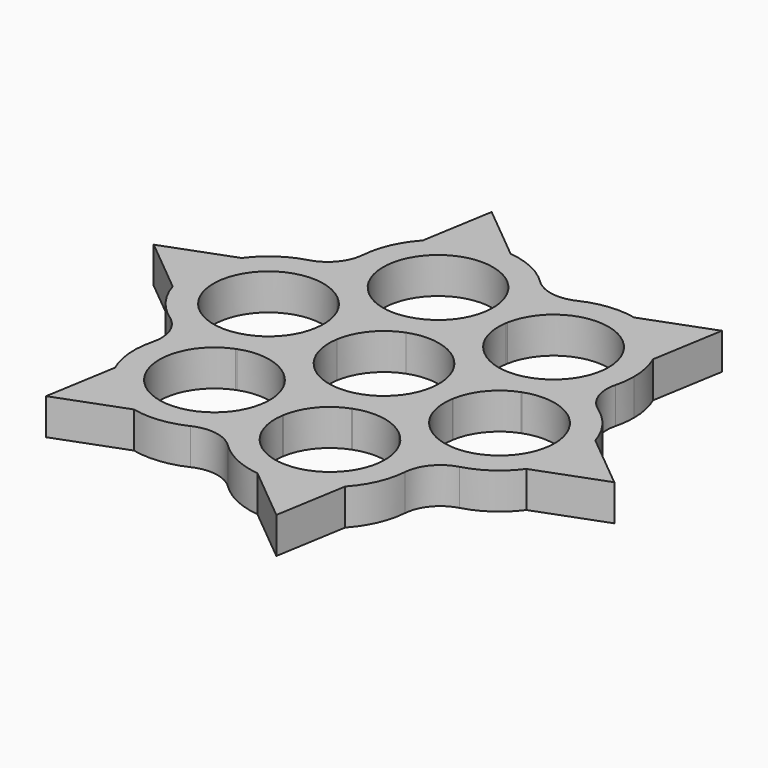
from build123d import *

# Parameters (mm, degrees)
F2_DEPTH    = 7.239
F3_DEPTH    = 7.239
F4_T1_DEPTH = 7.239
F5_R        = 7.62


# Not quite as in the source:
# - a fillet or chamfer that OpenCascade refuses, or shapes differently, is made with other operations: its cross-section is extruded or revolved along the edge and cut away or added


with BuildPart() as f2:
    # F0 (on Top) → F2 (new body)
    with BuildSketch(Plane.XY):
        with BuildLine():
            ThreePointArc((6.9968392918, 8.4855549709), (9.9476892075, 4.6908296356), (10.9982, 0))
            ThreePointArc((10.9982, 0), (10.9603663805, -0.9114669745), (10.8471258159, -1.8166630875))
            Line((10.8471258159, -1.8166630875), (15.8573455923, -2.6557684397))
            ThreePointArc((15.8573455923, -2.6557684397), (16.0228912675, -1.3324678865), (16.0782, 0))
            ThreePointArc((16.0782, 0), (14.542464823, 6.8574945943), (10.2286357315, 12.4049798997))
            Line((10.2286357315, 12.4049798997), (6.9968392918, 8.4855549709))
        make_face()
        with BuildLine():
            ThreePointArc((-3.8502865241, 10.3022180584), (1.8166630875, 10.8471258159), (6.9968392918, 8.4855549709))
            Line((6.9968392918, 8.4855549709), (10.2286357315, 12.4049798997))
            ThreePointArc((10.2286357315, 12.4049798997), (2.6557684397, 15.8573455923), (-5.6287098609, 15.0607483394))
            Line((-5.6287098609, 15.0607483394), (-3.8502865241, 10.3022180584))
        make_face()
        with BuildLine():
            Line((15.8573455923, -2.6557684397), (10.8471258159, -1.8166630875))
            ThreePointArc((10.8471258159, -1.8166630875), (8.4855549709, -6.9968392918), (3.8502865241, -10.3022180584))
            Line((3.8502865241, -10.3022180584), (5.6287098609, -15.0607483394))
            ThreePointArc((5.6287098609, -15.0607483394), (12.4049798997, -10.2286357315), (15.8573455923, -2.6557684397))
        make_face()
        with BuildLine():
            ThreePointArc((-10.8471258159, 1.8166630875), (-8.4855549709, 6.9968392918), (-3.8502865241, 10.3022180584))
            Line((-3.8502865241, 10.3022180584), (-5.6287098609, 15.0607483394))
            ThreePointArc((-5.6287098609, 15.0607483394), (-12.4049798997, 10.2286357315), (-15.8573455923, 2.6557684397))
            Line((-15.8573455923, 2.6557684397), (-10.8471258159, 1.8166630875))
        make_face()
        with BuildLine():
            Line((5.6287098609, -15.0607483394), (3.8502865241, -10.3022180584))
            ThreePointArc((3.8502865241, -10.3022180584), (-1.8166630875, -10.8471258159), (-6.9968392918, -8.4855549709))
            Line((-6.9968392918, -8.4855549709), (-10.2286357315, -12.4049798997))
            ThreePointArc((-10.2286357315, -12.4049798997), (-2.6557684397, -15.8573455923), (5.6287098609, -15.0607483394))
        make_face()
        with BuildLine():
            ThreePointArc((-6.9968392918, -8.4855549709), (-10.3022180584, -3.8502865241), (-10.8471258159, 1.8166630875))
            Line((-10.8471258159, 1.8166630875), (-15.8573455923, 2.6557684397))
            ThreePointArc((-15.8573455923, 2.6557684397), (-15.0607483394, -5.6287098609), (-10.2286357315, -12.4049798997))
            Line((-10.2286357315, -12.4049798997), (-6.9968392918, -8.4855549709))
        make_face()
    extrude(amount=F2_DEPTH)

    # F1 (on Top) → F3 (join)
    with BuildSketch(Plane.XY):
        with BuildLine():
            ThreePointArc((22.9514427755, 5.8656594668), (33.016468503, 4.5341364803), (37.7025851565, -4.4724170818))
            ThreePointArc((37.7025851565, -4.4724170818), (31.4379323636, -14.3998504902), (19.7807553883, -13.017810816))
            ThreePointArc((19.7807553883, -13.017810816), (22.8084512552, -16.3716447193), (24.7834468313, -20.4354528579))
            ThreePointArc((24.7834468313, -20.4354528579), (33.1080256386, -19.2203628308), (39.6794010209, -13.9675462837))
            ThreePointArc((39.6794010209, -13.9675462837), (41.9871109493, -9.4670950078), (42.7825851565, -4.4724170818))
            ThreePointArc((42.7825851565, -4.4724170818), (42.6022135722, -2.0708411606), (42.0651457783, 0.2768511103))
            ThreePointArc((42.0651457783, 0.2768511103), (37.5638328916, 7.3842650059), (30.0893074574, 11.2454331611))
            ThreePointArc((30.0893074574, 11.2454331611), (26.9017291405, 8.0495671456), (22.9514427755, 5.8656594668))
        make_face()
        with BuildLine():
            ThreePointArc((22.7561188104, 5.7926497032), (22.8536077582, 5.829617507), (22.9514427755, 5.8656594668))
            ThreePointArc((22.9514427755, 5.8656594668), (26.9017291405, 8.0495671456), (30.0893074574, 11.2454331611))
            ThreePointArc((30.0893074574, 11.2454331611), (25.5869892554, 11.5669077681), (21.1727380342, 10.624251271))
            ThreePointArc((21.1727380342, 10.624251271), (21.0752490864, 10.5872834672), (20.9774140691, 10.5512415074))
            ThreePointArc((20.9774140691, 10.5512415074), (17.0271277041, 8.3673338285), (13.8395493871, 5.1714678131))
            ThreePointArc((13.8395493871, 5.1714678131), (18.3418675892, 4.849993206), (22.7561188104, 5.7926497032))
        make_face()
        with BuildLine():
            ThreePointArc((24.7834468313, -20.4354528579), (22.8084512552, -16.3716447193), (19.7807553883, -13.017810816))
            ThreePointArc((19.7807553883, -13.017810816), (19.707218441, -12.957702062), (19.6342033145, -12.8969605092))
            ThreePointArc((19.6342033145, -12.8969605092), (15.7650750743, -10.5635101082), (11.3994817591, -9.3987186595))
            ThreePointArc((11.3994817591, -9.3987186595), (13.3744773351, -13.4625267981), (16.402173202, -16.8163607014))
            ThreePointArc((16.402173202, -16.8163607014), (16.4757101493, -16.8764694554), (16.5487252758, -16.9372110082))
            ThreePointArc((16.5487252758, -16.9372110082), (20.417853516, -19.2706614092), (24.7834468313, -20.4354528579))
        make_face()
        with BuildLine():
            ThreePointArc((21.1727380342, 10.624251271), (25.5869892554, 11.5669077681), (30.0893074574, 11.2454331611))
            ThreePointArc((30.0893074574, 11.2454331611), (32.4781911968, 15.8067442605), (33.302671688, 20.8893180559))
            ThreePointArc((33.302671688, 20.8893180559), (32.9570434325, 24.2051439777), (31.9350184005, 27.3784112637))
            ThreePointArc((31.9350184005, 27.3784112637), (27.4531526953, 33.294260623), (20.7917042689, 36.566797667))
            ThreePointArc((20.7917042689, 36.566797667), (12.3866178149, 36.2224092362), (5.3058447451, 31.6807427551))
            ThreePointArc((5.3058447451, 31.6807427551), (6.2730175907, 28.5865669578), (6.5998373584, 25.3612706897))
            ThreePointArc((6.5998373584, 25.3612706897), (6.5505250686, 24.1029885217), (6.4028906835, 22.852424727))
            ThreePointArc((6.4028906835, 22.852424727), (18.2099895812, 31.8432743148), (28.222671688, 20.8893180559))
            ThreePointArc((28.222671688, 20.8893180559), (26.2904582909, 14.6628993296), (21.1727380342, 10.624251271))
        make_face()
        with BuildLine():
            ThreePointArc((25.5567434338, -25.3617544356), (25.3622428304, -22.8684416359), (24.7834468313, -20.4354528579))
            ThreePointArc((24.7834468313, -20.4354528579), (20.417853516, -19.2706614092), (16.5487252758, -16.9372110082))
            ThreePointArc((16.5487252758, -16.9372110082), (19.4464839727, -20.7141136736), (20.4767434338, -25.3617544356))
            ThreePointArc((20.4767434338, -25.3617544356), (8.6144991811, -36.3259612364), (-1.3838939013, -23.6390071003))
            ThreePointArc((-1.3838939013, -23.6390071003), (-2.7742058336, -27.9382250388), (-5.3058324685, -31.6808322496))
            ThreePointArc((-5.3058324685, -31.6808322496), (-0.0911857517, -38.2818472587), (7.7431459541, -41.3460251674))
            ThreePointArc((7.7431459541, -41.3460251674), (15.1072895917, -40.4224892095), (21.2720483325, -36.289780673))
            ThreePointArc((21.2720483325, -36.289780673), (24.4472916397, -31.2307485904), (25.5567434338, -25.3617544356))
        make_face()
        with BuildLine():
            Line((53.2084477738, -8.9112843948), (42.0651457783, 0.2768511103))
            ThreePointArc((42.0651457783, 0.2768511103), (42.6022135722, -2.0708411606), (42.7825851565, -4.4724170818))
            ThreePointArc((42.7825851565, -4.4724170818), (41.9871109493, -9.4670950078), (39.6794010209, -13.9675462837))
            Line((39.6794010209, -13.9675462837), (53.2084477738, -8.9112843948))
        make_face()
        with BuildLine():
            ThreePointArc((1.3432183629, 23.3981640186), (1.2689892456, 18.9066190694), (2.4402643012, 14.5698459906))
            ThreePointArc((2.4402643012, 14.5698459906), (4.9605713467, 18.2883858101), (6.3537578179, 22.5590435404))
            ThreePointArc((6.3537578179, 22.5590435404), (6.3773323249, 22.7059002526), (6.4028906835, 22.852424727))
            ThreePointArc((6.4028906835, 22.852424727), (6.5505250686, 24.1029885217), (6.5998373584, 25.3612706897))
            ThreePointArc((6.5998373584, 25.3612706897), (6.2730175907, 28.5865669578), (5.3058447451, 31.6807427551))
            ThreePointArc((5.3058447451, 31.6807427551), (2.7855376997, 27.9622029355), (1.3923512285, 23.6915452052))
            ThreePointArc((1.3923512285, 23.6915452052), (1.3687767215, 23.544688493), (1.3432183629, 23.3981640186))
        make_face()
        with BuildLine():
            ThreePointArc((20.7917042689, 36.566797667), (27.4531526953, 33.294260623), (31.9350184005, 27.3784112637))
            Line((31.9350184005, 27.3784112637), (34.3206748537, 41.6230759294))
            Line((34.3206748537, 41.6230759294), (20.7917042689, 36.566797667))
        make_face()
        with BuildLine():
            ThreePointArc((-1.1472239849, -20.8904729728), (-1.4740007496, -17.6653867253), (-2.4410480826, -14.5713951588))
            ThreePointArc((-2.4410480826, -14.5713951588), (-4.9726747175, -18.3140023695), (-6.3629866498, -22.6132203081))
            ThreePointArc((-6.3629866498, -22.6132203081), (-6.3782276583, -22.7067149977), (-6.3942733749, -22.800074948))
            ThreePointArc((-6.3942733749, -22.800074948), (-6.4802418832, -27.317690643), (-5.3058324685, -31.6808322496))
            ThreePointArc((-5.3058324685, -31.6808322496), (-2.7742058336, -27.9382250388), (-1.3838939013, -23.6390071003))
            ThreePointArc((-1.3838939013, -23.6390071003), (-1.3686528928, -23.5455124107), (-1.3526071762, -23.4521524604))
            ThreePointArc((-1.3526071762, -23.4521524604), (-1.1986520321, -22.1754227824), (-1.1472239849, -20.8904729728))
        make_face()
        with BuildLine():
            Line((18.8864028853, -50.5343796221), (21.2720483325, -36.289780673))
            ThreePointArc((21.2720483325, -36.289780673), (15.1072895917, -40.4224892095), (7.7431459541, -41.3460251674))
            Line((7.7431459541, -41.3460251674), (18.8864028853, -50.5343796221))
        make_face()
        with BuildLine():
            ThreePointArc((-19.5826320581, 12.8547821817), (-15.7335197941, 10.5497372026), (-11.3973465236, 9.3979998437))
            ThreePointArc((-11.3973465236, 9.3979998437), (-13.3543168627, 13.4352222389), (-16.3506403955, 16.7745249899))
            ThreePointArc((-16.3506403955, 16.7745249899), (-16.4751157371, 16.8756446455), (-16.5981033888, 16.9785685637))
            ThreePointArc((-16.5981033888, 16.9785685637), (-20.4472156527, 19.2836135428), (-24.7833889233, 20.4353509017))
            ThreePointArc((-24.7833889233, 20.4353509017), (-22.8264185841, 16.3981285065), (-19.8300950513, 13.0588257555))
            ThreePointArc((-19.8300950513, 13.0588257555), (-19.7056197098, 12.9577060999), (-19.5826320581, 12.8547821817))
        make_face()
        with BuildLine():
            ThreePointArc((-20.9623218428, -10.5465860032), (-17.0201516931, -8.3639282637), (-13.8384771801, -5.173058854))
            ThreePointArc((-13.8384771801, -5.173058854), (-18.3329887567, -4.8504662547), (-22.74050602, -5.7877452262))
            ThreePointArc((-22.74050602, -5.7877452262), (-22.8527610261, -5.8303901525), (-22.9654749473, -5.8718069139))
            ThreePointArc((-22.9654749473, -5.8718069139), (-26.907645097, -8.0544646533), (-30.08931961, -11.2453340631))
            ThreePointArc((-30.08931961, -11.2453340631), (-25.5948080334, -11.5679266624), (-21.1872907701, -10.6306476908))
            ThreePointArc((-21.1872907701, -10.6306476908), (-21.075035764, -10.5880027646), (-20.9623218428, -10.5465860032))
        make_face()
        with BuildLine():
            ThreePointArc((1.5198373584, 25.3612706897), (1.4879195116, 24.5239780427), (1.3923512285, 23.6915452052))
            ThreePointArc((1.3923512285, 23.6915452052), (2.7855376997, 27.9622029355), (5.3058447451, 31.6807427551))
            ThreePointArc((5.3058447451, 31.6807427551), (0.091338843, 38.2813840303), (-7.742607452, 41.3455025812))
            ThreePointArc((-7.742607452, 41.3455025812), (-15.1070729788, 40.422018851), (-21.2720601129, 36.2890890994))
            ThreePointArc((-21.2720601129, 36.2890890994), (-25.1761478666, 28.8380586139), (-24.7833889233, 20.4353509017))
            ThreePointArc((-24.7833889233, 20.4353509017), (-20.4472156527, 19.2836135428), (-16.5981033888, 16.9785685637))
            ThreePointArc((-16.5981033888, 16.9785685637), (-14.0965912281, 35.3428721625), (1.5198373584, 25.3612706897))
        make_face()
        with BuildLine():
            ThreePointArc((-5.3058324685, -31.6808322496), (-6.4802418832, -27.317690643), (-6.3942733749, -22.800074948))
            ThreePointArc((-6.3942733749, -22.800074948), (-24.2125911511, -29.3839939289), (-21.1872907701, -10.6306476908))
            ThreePointArc((-21.1872907701, -10.6306476908), (-25.5948080334, -11.5679266624), (-30.08931961, -11.2453340631))
            ThreePointArc((-30.08931961, -11.2453340631), (-33.1993509809, -19.0623122674), (-31.9358563488, -27.3798253987))
            ThreePointArc((-31.9358563488, -27.3798253987), (-27.4539661915, -33.2955299887), (-20.7925819899, -36.5679695525))
            ThreePointArc((-20.7925819899, -36.5679695525), (-12.3868483531, -36.2233364071), (-5.3058324685, -31.6808322496))
        make_face()
        with BuildLine():
            ThreePointArc((-22.9654749473, -5.8718069139), (-37.5527582872, 6.269171632), (-19.8300950513, 13.0588257555))
            ThreePointArc((-19.8300950513, 13.0588257555), (-22.8264185841, 16.3981285065), (-24.7833889233, 20.4353509017))
            ThreePointArc((-24.7833889233, 20.4353509017), (-33.1068810285, 19.2196489963), (-39.6773435015, 13.967270979))
            ThreePointArc((-39.6773435015, 13.967270979), (-42.5597216901, 7.1278288359), (-42.0630271426, -0.277531883))
            ThreePointArc((-42.0630271426, -0.277531883), (-37.5624514565, -7.3840241497), (-30.08931961, -11.2453340631))
            ThreePointArc((-30.08931961, -11.2453340631), (-26.907645097, -8.0544646533), (-22.9654749473, -5.8718069139))
        make_face()
        with BuildLine():
            ThreePointArc((-21.2720601129, 36.2890890994), (-15.1070729788, 40.422018851), (-7.742607452, 41.3455025812))
            Line((-7.742607452, 41.3455025812), (-18.8862220931, 50.5338958762))
            Line((-18.8862220931, 50.5338958762), (-21.2720601129, 36.2890890994))
        make_face()
        with BuildLine():
            Line((-34.3216271506, -41.6242308463), (-20.7925819899, -36.5679695525))
            ThreePointArc((-20.7925819899, -36.5679695525), (-27.4539661915, -33.2955299887), (-31.9358563488, -27.3798253987))
            Line((-31.9358563488, -27.3798253987), (-34.3216271506, -41.6242308463))
        make_face()
        with BuildLine():
            ThreePointArc((-42.0630271426, -0.277531883), (-42.5597216901, 7.1278288359), (-39.6773435015, 13.967270979))
            Line((-39.6773435015, 13.967270979), (-53.2064354224, 8.9109473688))
            Line((-53.2064354224, 8.9109473688), (-42.0630271426, -0.277531883))
        make_face()
    extrude(amount=F3_DEPTH)

    # F4: fillet of radius 10.795 on 12 edges, made by hand

    # F4_s2 → F4_t1 (join)
    with BuildSketch(Plane.XY):
        with BuildLine():
            ThreePointArc((-1.3526071762, -23.4521524604), (0.9769559698, -18.3362457073), (5.5628184207, -15.0852101894))
            ThreePointArc((5.5628184207, -15.0852101894), (1.8731173949, -15.9687177464), (-1.9208840616, -15.963042306))
            ThreePointArc((-1.9208840616, -15.963042306), (-1.1933128973, -19.6739495184), (-1.3526071762, -23.4521524604))
        make_face()
        with BuildLine():
            ThreePointArc((-6.3629866498, -22.6132203081), (-6.8983359675, -17.0173110878), (-10.1746370694, -12.4493082437))
            ThreePointArc((-10.1746370694, -12.4493082437), (-6.9745076224, -14.4867097253), (-3.3860894153, -15.7175988532))
            ThreePointArc((-3.3860894153, -15.7175988532), (-5.2828367995, -18.9891436011), (-6.3629866498, -22.6132203081))
        make_face()
        with BuildLine():
            ThreePointArc((-22.74050602, -5.7877452262), (-18.1782362606, -2.5250489433), (-15.8688205194, 2.5863198877))
            ThreePointArc((-15.8688205194, 2.5863198877), (-16.0330506196, -1.2040776835), (-15.3045399233, -4.9274306668))
            ThreePointArc((-15.3045399233, -4.9274306668), (-19.0732876307, -4.9188132222), (-22.74050602, -5.7877452262))
        make_face()
        with BuildLine():
            ThreePointArc((1.3432183629, 23.3981640186), (-0.9946746618, 18.3151486302), (-5.5630223933, 15.0851349709))
            ThreePointArc((-5.5630223933, 15.0851349709), (-1.8739143008, 15.9686242499), (1.9195066472, 15.9632079944))
            ThreePointArc((1.9195066472, 15.9632079944), (1.1943532617, 19.6468131354), (1.3432183629, 23.3981640186))
        make_face()
        with BuildLine():
            ThreePointArc((20.9774140691, 10.5512415074), (15.3864187742, 10.014970975), (10.2827878764, 12.3601289932))
            ThreePointArc((10.2827878764, 12.3601289932), (12.8927630235, 9.6065174158), (14.7848395574, 6.3179929173))
            ThreePointArc((14.7848395574, 6.3179929173), (17.6307978726, 8.8008089406), (20.9774140691, 10.5512415074))
        make_face()
        with BuildLine():
            ThreePointArc((19.6342033145, -12.8969605092), (16.3683528699, -8.3216300638), (15.8456559401, -2.7246473292))
            ThreePointArc((15.8456559401, -2.7246473292), (14.7661799124, -6.3614814339), (12.8646328491, -9.6441555824))
            ThreePointArc((12.8646328491, -9.6441555824), (16.4420144413, -10.8697363992), (19.6342033145, -12.8969605092))
        make_face()
        with BuildLine():
            ThreePointArc((-20.9623218428, -10.5465860032), (-15.3782970714, -10.0168926157), (-10.2822955556, -12.3605385541))
            ThreePointArc((-10.2822955556, -12.3605385541), (-12.8920067418, -9.6075323268), (-14.7840963785, -6.3197317595))
            ThreePointArc((-14.7840963785, -6.3197317595), (-17.6237877974, -8.7977281379), (-20.9623218428, -10.5465860032))
        make_face()
        with BuildLine():
            ThreePointArc((16.402173202, -16.8163607014), (11.288380593, -14.4824521842), (5.6944920196, -15.0359993309))
            ThreePointArc((5.6944920196, -15.0359993309), (9.0592404484, -13.2830221613), (11.9195455992, -10.7904099991))
            ThreePointArc((11.9195455992, -10.7904099991), (13.8040728015, -14.0687943349), (16.402173202, -16.8163607014))
        make_face()
        with BuildLine():
            ThreePointArc((22.7561188104, 5.7926497032), (18.1835455392, 2.5307260226), (15.8687246761, -2.5869078828))
            ThreePointArc((15.8687246761, -2.5869078828), (16.0331248451, 1.203088916), (15.3049650408, 4.9261100616))
            ThreePointArc((15.3049650408, 4.9261100616), (19.0817849197, 4.9187544216), (22.7561188104, 5.7926497032))
        make_face()
        with BuildLine():
            ThreePointArc((6.3537578179, 22.5590435404), (6.9078909376, 16.9916383529), (10.17454185, 12.4493860644))
            ThreePointArc((10.17454185, 12.4493860644), (6.9746678336, 14.4866325918), (3.3865572791, 15.7174980527))
            ThreePointArc((3.3865572791, 15.7174980527), (5.2722887952, 18.9638651664), (6.3537578179, 22.5590435404))
        make_face()
        with BuildLine():
            ThreePointArc((-16.3506403955, 16.7745249899), (-11.2553865221, 14.4772739198), (-5.6942102807, 15.0361060291))
            ThreePointArc((-5.6942102807, 15.0361060291), (-9.0583348552, 13.2836397456), (-11.9182764268, 10.7918118152))
            ThreePointArc((-11.9182764268, 10.7918118152), (-13.78336795, 14.0432779322), (-16.3506403955, 16.7745249899))
        make_face()
        with BuildLine():
            ThreePointArc((-19.5826320581, 12.8547821817), (-16.3566495613, 8.2906133369), (-15.8456168312, 2.724874764))
            ThreePointArc((-15.8456168312, 2.724874764), (-14.7662289393, 6.3613676321), (-12.8649199207, 9.643772637))
            ThreePointArc((-12.8649199207, 9.643772637), (-16.4122105492, 10.8550558687), (-19.5826320581, 12.8547821817))
        make_face()
    extrude(amount=F4_T1_DEPTH)

    # F5
    f5_edges = [f2.edges().sort_by_distance(p)[0] for p in [
        (5.305845, 31.680743, 3.6195),
        (30.089307, 11.245433, 3.6195),
        (-30.08932, -11.245334, 3.6195),
        (-5.305832, -31.680832, 3.6195),
        (24.783447, -20.435453, 3.6195),
        (-24.783389, 20.435351, 3.6195),
    ]]
    fillet(f5_edges, radius=F5_R)


solid = f2.part
